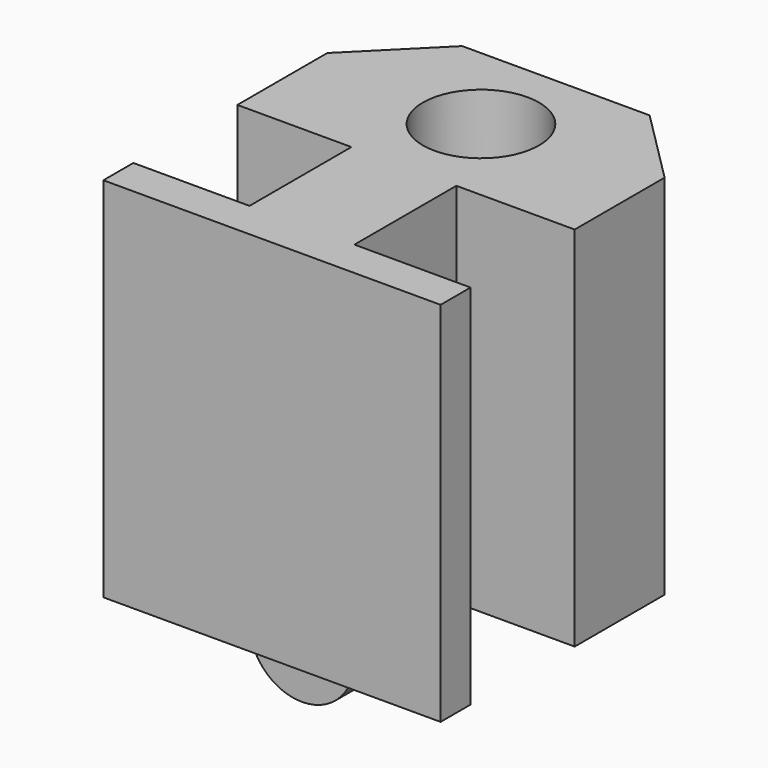
from build123d import *

# Parameters (mm, degrees)
F1_DEPTH    = 3.4
F2_W        = 9
F2_H        = 9.8
F3_DEPTH    = 1
F4_W        = 9.0031104628
F4_H        = 9.8
F5_DEPTH    = 5
F7_D        = 3.1
F8_T1_DEPTH = 20.0867319519
F8_T3_DEPTH = 19.2898424147


# Not quite as in the source:
# - a fillet or chamfer that OpenCascade refuses, or shapes differently, is made with other operations: its cross-section is extruded or revolved along the edge and cut away or added


with BuildPart() as f1:
    # F0 (on Front) → F1 (new body)
    with BuildSketch(Plane.XZ):
        with BuildLine():
            Line((2.8, 0), (0, 0))
            Line((0, 0), (0, -9.8))
            ThreePointArc((0, -9.8), (1.4, -11.2), (2.8, -9.8))
            Line((2.8, -9.8), (2.8, 0))
        make_face()
    extrude(amount=F1_DEPTH)

    # F2 (on face) → F3 (join)
    with BuildSketch(Plane.XZ.offset(3.4)):
        with Locations((1.4, -4.9)):
            Rectangle(F2_W, F2_H)
    extrude(amount=F3_DEPTH)

    # F4 (on face) → F5 (join)
    with BuildSketch(Plane(origin=(0, 0, 0), x_dir=(-1, 0, 0), z_dir=(0, 1, 0))):
        with Locations((-1.4576160967, -4.9)):
            Rectangle(F4_W, F4_H)
    extrude(amount=F5_DEPTH)

    # F7 (through all)
    with Locations(Plane.XY):
        with Locations((1.4576160967, 2.5)):
            Hole(F7_D / 2)

    # F8: chamfer of 2 on 3 edges, made by hand

    # F8_s2 → F8_t1 (cut)
    with BuildSketch(Plane.XY.offset(-14.9433659759)):
        Polygon((-1.0439391347, 5), (-3.0439391347, 3), (-3.0439391347, 5), align=None)
        Polygon((5.9591713281, 3), (3.9591713281, 5), (5.9591713281, 5), align=None)
    extrude(amount=F8_T1_DEPTH, mode=Mode.SUBTRACT)

    # F8_s4 → F8_t3 (cut)
    with BuildSketch(Plane.YZ.offset(-8.1873051107)):
        Polygon((5, -7.8), (3, -9.8), (5, -9.8), align=None)
    extrude(amount=F8_T3_DEPTH, mode=Mode.SUBTRACT)


solid = f1.part
